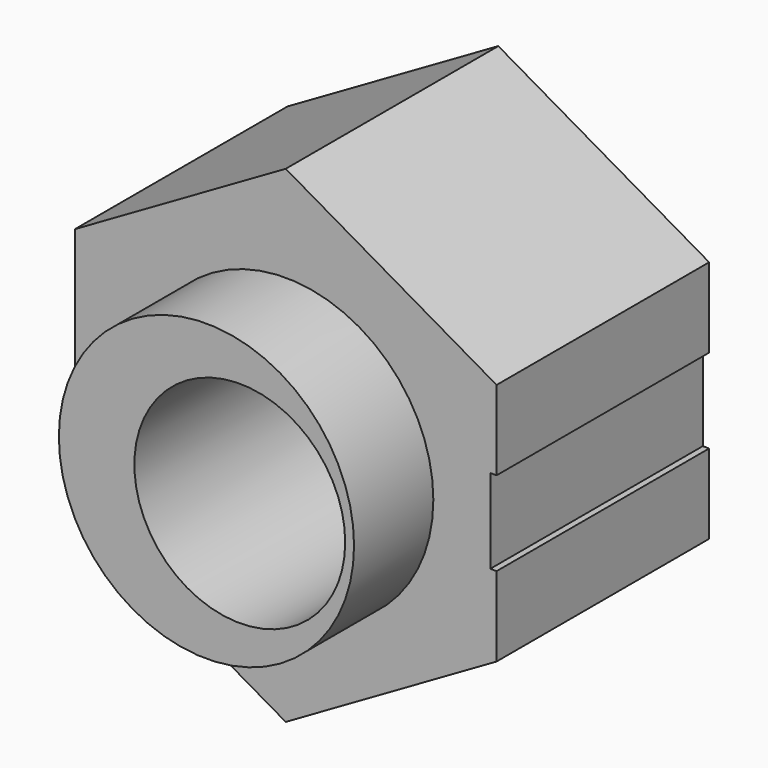
from build123d import *

# Parameters (mm, degrees)
F0_R     = 2.5
F1_DEPTH = 6.3
F3_R     = 3.5
F4_DEPTH = 2.35
F5_DEPTH = 8.65
F0_W     = 0.15
F0_H     = 2
F8_DEPTH = 22


# Not quite as in the source:
# - an extrude ends at something that could not be found from the text; its depth is read off the source's solid
# - a feature names something its author has since deleted; it is built from what else it names


with BuildPart() as f1:
    # F0 (on Front) → F1 (new body)
    with BuildSketch(Plane.XZ):
        Polygon((5, 1), (5, 2.8867513459), (0, 5.7735026919), (-5, 2.8867513459), (-5, -2.8867513459), (0, -5.7735026919), (5, -2.8867513459), (5, -1), (4.85, -1), (4.85, 1), align=None)
        with Locations((0.79, 0)):
            Circle(F0_R, mode=Mode.SUBTRACT)
    extrude(amount=F1_DEPTH)

    # F3 (on offset) → F4 (join)
    with BuildSketch(Plane.XZ.offset(6.3)):
        Circle(F3_R)
    extrude(amount=F4_DEPTH)

    # F0 (on Front) → F5 (cut, through all)
    with BuildSketch(Plane.XZ):
        with Locations((0.79, 0)):
            Circle(F0_R)
    extrude(amount=F5_DEPTH, mode=Mode.SUBTRACT)

    # F6 (on Top) → F7 (revolve, cut)
    with BuildSketch(Plane.XY):
        Polygon((-6.0966597098, -6.5938490836), (-5, -6.3), (-6.0966597098, -6.3), align=None)
    revolve(axis=Axis((0, -6.5372320823, 0), (0, -1, 0)), mode=Mode.SUBTRACT)

    # F0 (on Front) → F8 (cut, through all)
    with BuildSketch(Plane.XZ):
        with Locations((4.925, 0)):
            Rectangle(F0_W, F0_H)
    extrude(amount=-F8_DEPTH, mode=Mode.SUBTRACT)


solid = f1.part
